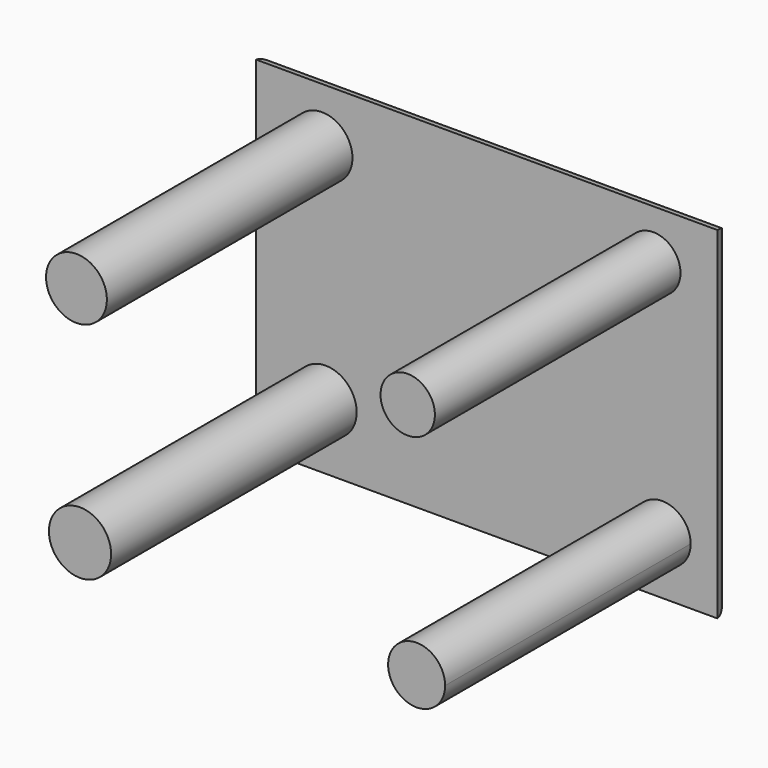
from build123d import *

# Parameters (mm, degrees)
F0_R        = 6.9755689081
F1_DEPTH    = 70.358
F0_R_2      = 7.1291532236
F0_R_3      = 6.2311216895
F2_W        = 105.7274974883
F2_H        = 78.3771444112
F3_DEPTH    = 4.572
F4_T1_DEPTH = 131.0001783908
F4_T3_DEPTH = 103.6498253137


# Not quite as in the source:
# - a fillet or chamfer that OpenCascade refuses, or shapes differently, is made with other operations: its cross-section is extruded or revolved along the edge and cut away or added


with BuildPart() as f1:
    # F0 (on Front) → F1 (new body)
    with BuildSketch(Plane.XZ):
        with Locations((-14.6957142279, 3.8780358154)):
            Circle(F0_R)
    extrude(amount=F1_DEPTH)


with BuildPart() as f1b:
    # F0 (on Front) → F1, piece 2 (new body)
    with BuildSketch(Plane.XZ):
        with Locations((-13.8792861253, -47.1487529576)):
            Circle(F0_R_2)
    extrude(amount=F1_DEPTH)


with BuildPart() as f1c:
    # F0 (on Front) → F1, piece 3 (new body)
    with BuildSketch(Plane.XZ):
        with Locations((61.2321421504, 5.1026786678)):
            Circle(F0_R_3)
    extrude(amount=F1_DEPTH)


with BuildPart() as f1d:
    # F0 (on Front) → F1, piece 4 (new body)
    with BuildSketch(Plane.XZ):
        with BuildLine():
            ThreePointArc((69.8046460748, -48.7816073), (58.6547937541, -44.1631872504), (63.2732138038, -55.313039571))
            ThreePointArc((63.2732138038, -55.313039571), (67.8916338535, -53.4000273497), (69.8046460748, -48.7816073))
        make_face()
    extrude(amount=F1_DEPTH)


with BuildPart() as f3:
    # F2 (on Front) → F3 (new body)
    with BuildSketch(Plane.XZ):
        with Locations((23.0641048402, -22.6558921859)):
            Rectangle(F2_W, F2_H)
    extrude(amount=-F3_DEPTH)

    # F4: fillet of radius 5.08 on 4 edges, made by hand

    # F4_s2 → F4_t1 (cut)
    with BuildSketch(Plane.YZ.offset(-42.4359843552)):
        with BuildLine():
            ThreePointArc((0, 16.5326800197), (3.2594288314, 14.8859114369), (4.572, 11.4781438392))
            Line((4.572, 11.4781438392), (4.572, 16.5326800197))
            Line((4.572, 16.5326800197), (0, 16.5326800197))
        make_face()
        with BuildLine():
            ThreePointArc((0, -61.8444643915), (3.2594288314, -60.1976958087), (4.572, -56.789928211))
            Line((4.572, -56.789928211), (4.572, -61.8444643915))
            Line((4.572, -61.8444643915), (0, -61.8444643915))
        make_face()
    extrude(amount=F4_T1_DEPTH, mode=Mode.SUBTRACT)

    # F4_s4 → F4_t3 (cut)
    with BuildSketch(Plane.XY.offset(-74.4808048427)):
        with BuildLine():
            ThreePointArc((75.9278535843, 0), (74.2810850015, 3.2594288314), (70.8733174038, 4.572))
            Line((70.8733174038, 4.572), (75.9278535843, 4.572))
            Line((75.9278535843, 4.572), (75.9278535843, 0))
        make_face()
        with BuildLine():
            ThreePointArc((-29.799643904, 0), (-28.1528753212, 3.2594288314), (-24.7451077235, 4.572))
            Line((-24.7451077235, 4.572), (-29.799643904, 4.572))
            Line((-29.799643904, 4.572), (-29.799643904, 0))
        make_face()
    extrude(amount=F4_T3_DEPTH, mode=Mode.SUBTRACT)


solid = Compound([f1.part, f1b.part, f1c.part, f1d.part, f3.part])
